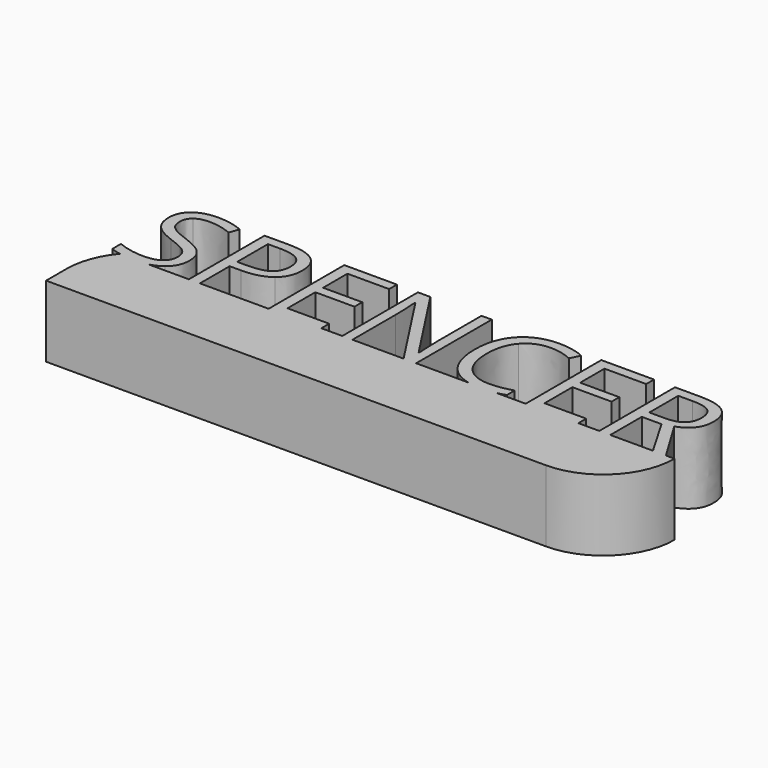
from build123d import *

# Parameters (mm, degrees)
F1_DEPTH    = 15
F2_T1_DEPTH = 63.1127871351
F2_T3_DEPTH = 90


# Not quite as in the source:
# - a fillet or chamfer that OpenCascade refuses, or shapes differently, is made with other operations: its cross-section is extruded or revolved along the edge and cut away or added


with BuildPart() as f1:
    # F0 (on Top) → F1 (new body)
    with BuildSketch(Plane.XY):
        with BuildLine():
            Line((-120, 0), (0, 0))
            Line((0, 0), (0, 15))
            Line((0, 15), (-1.8037596436, 15))
            Line((-1.8037596436, 15), (-4.5333043573, 15))
            Line((-4.5333043573, 15), (-13.4869064436, 15))
            Line((-13.4869064436, 15), (-15.7948495056, 15))
            Line((-15.7948495056, 15), (-20.1934151907, 15))
            Line((-20.1934151907, 15), (-31.2637183527, 15))
            Line((-31.2637183527, 15), (-37.436193108, 15))
            add(Edge.make_bspline(
                [(-37.436193108, 15), (-38.8938347302, 14.7261762469), (-40.691078996, 14.7261762469)],
                knots=[0.406741787, 0.406741787, 0.406741787, 1, 1, 1], degree=2))
            add(Edge.make_bspline(
                [(-40.691078996, 14.7261762469), (-42.097002764, 14.7261762469), (-43.2972236962, 15)],
                knots=[0, 0, 0, 0.3205826669, 0.3205826669, 0.3205826669], degree=2))
            Line((-43.2972236962, 15), (-54.2736064327, 15))
            Line((-54.2736064327, 15), (-56.9075301532, 15))
            Line((-56.9075301532, 15), (-67.6518526567, 15))
            Line((-67.6518526567, 15), (-69.7859393676, 15))
            Line((-69.7859393676, 15), (-74.1845050527, 15))
            Line((-74.1845050527, 15), (-85.2548082147, 15))
            Line((-85.2548082147, 15), (-99.693578181, 15))
            Line((-99.693578181, 15), (-102.0015212431, 15))
            Line((-102.0015212431, 15), (-110.5667825436, 15))
            add(Edge.make_bspline(
                [(-110.5667825436, 15), (-111.7209724053, 14.7261762469), (-113.1283277192, 14.7261762469)],
                knots=[0.5682703015, 0.5682703015, 0.5682703015, 1, 1, 1], degree=2))
            add(Edge.make_bspline(
                [(-113.1283277192, 14.7261762469), (-115.0613961391, 14.7261762469), (-116.5067974938, 15)],
                knots=[0, 0, 0, 0.5477225575, 0.5477225575, 0.5477225575], degree=2))
            Line((-116.5067974938, 15), (-120, 15))
            Line((-120, 15), (-120, 0))
        make_face()
        with BuildLine():
            Line((-4.5333043573, 15), (-1.8037596436, 15))
            Line((-1.8037596436, 15), (-7.1976529393, 23.9231772248))
            add(Edge.make_bspline(
                [(-3.2033032707, 29.24752798), (-3.2033032707, 25.3096816256), (-7.1976529393, 23.9231772248)],
                knots=[0, 0, 0, 1, 1, 1], degree=2))
            add(Edge.make_bspline(
                [(-4.9483863957, 33.4591980876), (-3.2033032707, 32.0596544605), (-3.2033032707, 29.24752798)],
                knots=[0, 0, 0, 1, 1, 1], degree=2))
            add(Edge.make_bspline(
                [(-10.3487993046, 34.8587417147), (-6.6934695208, 34.8587417147), (-4.9483863957, 33.4591980876)],
                knots=[0, 0, 0, 1, 1, 1], degree=2))
            Line((-10.3487993046, 34.8587417147), (-15.7948495056, 34.8587417147))
            Line((-15.7948495056, 34.8587417147), (-15.7948495056, 15))
            Line((-15.7948495056, 15), (-13.4869064436, 15))
            Line((-13.4869064436, 15), (-13.4869064436, 23.2581766815))
            Line((-13.4869064436, 23.2581766815), (-9.3404324677, 23.2581766815))
            Line((-9.3404324677, 23.2581766815), (-4.5333043573, 15))
        make_face()
        with BuildLine():
            Line((-10.3183744431, 25.2401390851), (-13.4869064436, 25.2401390851))
            Line((-13.4869064436, 25.2401390851), (-13.4869064436, 32.8333152233))
            Line((-13.4869064436, 32.8333152233), (-10.4835379767, 32.8333152233))
            add(Edge.make_bspline(
                [(-6.7543192437, 31.9640334673), (-7.9148103879, 32.8333152233), (-10.4835379767, 32.8333152233)],
                knots=[0, 0, 0, 1, 1, 1], degree=2))
            add(Edge.make_bspline(
                [(-5.5938280995, 29.1258285342), (-5.5938280995, 31.0947517114), (-6.7543192437, 31.9640334673)],
                knots=[0, 0, 0, 1, 1, 1], degree=2))
            add(Edge.make_bspline(
                [(-6.7347604042, 26.2115614474), (-5.5938280995, 27.1829838096), (-5.5938280995, 29.1258285342)],
                knots=[0, 0, 0, 1, 1, 1], degree=2))
            add(Edge.make_bspline(
                [(-10.3183744431, 25.2401390851), (-7.8756927089, 25.2401390851), (-6.7347604042, 26.2115614474)],
                knots=[0, 0, 0, 1, 1, 1], degree=2))
        make_face(mode=Mode.SUBTRACT)
        with BuildLine():
            add(Edge.make_bspline(
                [(-116.5067974938, 15), (-117.7003258945, 15.2261077348), (-118.5613386939, 15.6389220906)],
                knots=[0.5477225575, 0.5477225575, 0.5477225575, 1, 1, 1], degree=2))
            Line((-116.5067974938, 15), (-110.5667825436, 15))
            add(Edge.make_bspline(
                [(-107.9669672933, 16.1952624144), (-109.0475638679, 15.360424375), (-110.5667825436, 15)],
                knots=[0, 0, 0, 0.5682703015, 0.5682703015, 0.5682703015], degree=2))
            add(Edge.make_bspline(
                [(-106.0654134521, 20.2852330762), (-106.0654134521, 17.664348582), (-107.9669672933, 16.1952624144)],
                knots=[0, 0, 0, 1, 1, 1], degree=2))
            add(Edge.make_bspline(
                [(-107.2389438227, 23.5971965663), (-106.0654134521, 22.3193523851), (-106.0654134521, 20.2852330762)],
                knots=[0, 0, 0, 1, 1, 1], degree=2))
            add(Edge.make_bspline(
                [(-111.5375421058, 25.9877213952), (-108.4124741932, 24.8750407476), (-107.2389438227, 23.5971965663)],
                knots=[0, 0, 0, 1, 1, 1], degree=2))
            add(Edge.make_bspline(
                [(-114.3018580898, 27.2025426491), (-113.3978050636, 26.6527219385), (-111.5375421058, 25.9877213952)],
                knots=[0, 0, 0, 1, 1, 1], degree=2))
            add(Edge.make_bspline(
                [(-115.5862218842, 28.4130174943), (-115.2059111159, 27.7523633598), (-114.3018580898, 27.2025426491)],
                knots=[0, 0, 0, 1, 1, 1], degree=2))
            add(Edge.make_bspline(
                [(-115.9665326524, 30.1037705096), (-115.9665326524, 29.0736716288), (-115.5862218842, 28.4130174943)],
                knots=[0, 0, 0, 1, 1, 1], degree=2))
            add(Edge.make_bspline(
                [(-114.9342605672, 32.2900141258), (-115.9665326524, 31.5033141367), (-115.9665326524, 30.1037705096)],
                knots=[0, 0, 0, 1, 1, 1], degree=2))
            add(Edge.make_bspline(
                [(-112.067803977, 33.076714115), (-113.901988482, 33.076714115), (-114.9342605672, 32.2900141258)],
                knots=[0, 0, 0, 1, 1, 1], degree=2))
            add(Edge.make_bspline(
                [(-107.2867543192, 32.0466152342), (-109.7468216886, 33.076714115), (-112.067803977, 33.076714115)],
                knots=[0, 0, 0, 1, 1, 1], degree=2))
            Line((-107.2867543192, 32.0466152342), (-106.5652504618, 34.0546560904))
            add(Edge.make_bspline(
                [(-112.0113006628, 35.1412582853), (-109.0513962838, 35.1412582853), (-106.5652504618, 34.0546560904)],
                knots=[0, 0, 0, 1, 1, 1], degree=2))
            add(Edge.make_bspline(
                [(-116.577203086, 33.7830055417), (-114.8538520048, 35.1412582853), (-112.0113006628, 35.1412582853)],
                knots=[0, 0, 0, 1, 1, 1], degree=2))
            add(Edge.make_bspline(
                [(-118.3005541671, 30.1298489623), (-118.3005541671, 32.424752798), (-116.577203086, 33.7830055417)],
                knots=[0, 0, 0, 1, 1, 1], degree=2))
            add(Edge.make_bspline(
                [(-117.1118113659, 26.5853526024), (-118.3005541671, 27.9436053461), (-118.3005541671, 30.1298489623)],
                knots=[0, 0, 0, 1, 1, 1], degree=2))
            add(Edge.make_bspline(
                [(-113.1544061719, 24.236118657), (-115.9230685646, 25.2270998587), (-117.1118113659, 26.5853526024)],
                knots=[0, 0, 0, 1, 1, 1], degree=2))
            add(Edge.make_bspline(
                [(-110.2010214061, 22.9734869064), (-111.1724437683, 23.5320004346), (-113.1544061719, 24.236118657)],
                knots=[0, 0, 0, 1, 1, 1], degree=2))
            add(Edge.make_bspline(
                [(-108.8145170053, 21.7564924481), (-109.2295990438, 22.4149733782), (-110.2010214061, 22.9734869064)],
                knots=[0, 0, 0, 1, 1, 1], degree=2))
            add(Edge.make_bspline(
                [(-108.3994349669, 20.0679126372), (-108.3994349669, 21.098011518), (-108.8145170053, 21.7564924481)],
                knots=[0, 0, 0, 1, 1, 1], degree=2))
            add(Edge.make_bspline(
                [(-109.5686189286, 17.6274041074), (-108.3994349669, 18.5032054765), (-108.3994349669, 20.0679126372)],
                knots=[0, 0, 0, 1, 1, 1], degree=2))
            add(Edge.make_bspline(
                [(-113.0457459524, 16.7516027382), (-110.7378028904, 16.7516027382), (-109.5686189286, 17.6274041074)],
                knots=[0, 0, 0, 1, 1, 1], degree=2))
            add(Edge.make_bspline(
                [(-115.8969901119, 17.051504944), (-114.4583288058, 16.7516027382), (-113.0457459524, 16.7516027382)],
                knots=[0, 0, 0, 1, 1, 1], degree=2))
            add(Edge.make_bspline(
                [(-118.5613386939, 17.8642833859), (-117.335651418, 17.3514071498), (-115.8969901119, 17.051504944)],
                knots=[0, 0, 0, 1, 1, 1], degree=2))
            Line((-118.5613386939, 17.8642833859), (-118.5613386939, 15.6389220906))
        make_face()
        with BuildLine():
            Line((-110.5667825436, 15), (-116.5067974938, 15))
            add(Edge.make_bspline(
                [(-113.1283277192, 14.7261762469), (-115.0613961391, 14.7261762469), (-116.5067974938, 15)],
                knots=[0, 0, 0, 0.5477225575, 0.5477225575, 0.5477225575], degree=2))
            add(Edge.make_bspline(
                [(-110.5667825436, 15), (-111.7209724053, 14.7261762469), (-113.1283277192, 14.7261762469)],
                knots=[0.5682703015, 0.5682703015, 0.5682703015, 1, 1, 1], degree=2))
        make_face()
        with BuildLine():
            Line((-102.0015212431, 34.8587417147), (-102.0015212431, 15))
            Line((-102.0015212431, 15), (-99.693578181, 15))
            Line((-99.693578181, 15), (-99.693578181, 22.8104965772))
            Line((-99.693578181, 22.8104965772), (-97.3552102575, 22.8104965772))
            add(Edge.make_bspline(
                [(-91.4679995654, 24.4338802564), (-93.5260241226, 22.8104965772), (-97.3552102575, 22.8104965772)],
                knots=[0, 0, 0, 1, 1, 1], degree=2))
            add(Edge.make_bspline(
                [(-89.4099750081, 29.0736716288), (-89.4099750081, 26.0572639357), (-91.4679995654, 24.4338802564)],
                knots=[0, 0, 0, 1, 1, 1], degree=2))
            add(Edge.make_bspline(
                [(-96.8510268391, 34.8587417147), (-89.4099750081, 34.8587417147), (-89.4099750081, 29.0736716288)],
                knots=[0, 0, 0, 1, 1, 1], degree=2))
            Line((-96.8510268391, 34.8587417147), (-102.0015212431, 34.8587417147))
        make_face()
        with BuildLine():
            Line((-97.6116483755, 24.7924589808), (-99.693578181, 24.7924589808))
            Line((-99.693578181, 24.7924589808), (-99.693578181, 32.859393676))
            Line((-99.693578181, 32.859393676), (-97.1118113659, 32.859393676))
            add(Edge.make_bspline(
                [(-93.0913832446, 31.8966641313), (-94.3822666522, 32.859393676), (-97.1118113659, 32.859393676)],
                knots=[0, 0, 0, 1, 1, 1], degree=2))
            add(Edge.make_bspline(
                [(-91.800499837, 28.9650114093), (-91.800499837, 30.9339345865), (-93.0913832446, 31.8966641313)],
                knots=[0, 0, 0, 1, 1, 1], degree=2))
            add(Edge.make_bspline(
                [(-93.171791807, 25.7834401825), (-91.800499837, 26.7744213843), (-91.800499837, 28.9650114093)],
                knots=[0, 0, 0, 1, 1, 1], degree=2))
            add(Edge.make_bspline(
                [(-97.6116483755, 24.7924589808), (-94.543083777, 24.7924589808), (-93.171791807, 25.7834401825)],
                knots=[0, 0, 0, 1, 1, 1], degree=2))
        make_face(mode=Mode.SUBTRACT)
        Polygon((-31.2637183527, 15), (-20.1934151907, 15), (-20.1934151907, 17.0645441704), (-28.9557752907, 17.0645441704), (-28.9557752907, 24.3708573291), (-20.7236770618, 24.3708573291), (-20.7236770618, 26.4093230468), (-28.9557752907, 26.4093230468), (-28.9557752907, 32.8072367706), (-20.1934151907, 32.8072367706), (-20.1934151907, 34.8587417147), (-31.2637183527, 34.8587417147), align=None)
        Polygon((-85.2548082147, 34.8587417147), (-85.2548082147, 15), (-74.1845050527, 15), (-74.1845050527, 17.0645441704), (-82.9468651527, 17.0645441704), (-82.9468651527, 24.3708573291), (-74.7147669238, 24.3708573291), (-74.7147669238, 26.4093230468), (-82.9468651527, 26.4093230468), (-82.9468651527, 32.8072367706), (-74.1845050527, 32.8072367706), (-74.1845050527, 34.8587417147), align=None)
        with BuildLine():
            add(Edge.make_bspline(
                [(-37.436193108, 15), (-38.8938347302, 14.7261762469), (-40.691078996, 14.7261762469)],
                knots=[0.406741787, 0.406741787, 0.406741787, 1, 1, 1], degree=2))
            Line((-37.436193108, 15), (-43.2972236962, 15))
            add(Edge.make_bspline(
                [(-40.691078996, 14.7261762469), (-42.097002764, 14.7261762469), (-43.2972236962, 15)],
                knots=[0, 0, 0, 0.3205826669, 0.3205826669, 0.3205826669], degree=2))
        make_face()
        with BuildLine():
            Line((-43.2972236962, 15), (-37.436193108, 15))
            add(Edge.make_bspline(
                [(-35.5970879061, 15.5041834185), (-36.4368242914, 15.1877353912), (-37.436193108, 15)],
                knots=[0, 0, 0, 0.406741787, 0.406741787, 0.406741787], degree=2))
            Line((-35.5970879061, 15.5041834185), (-35.5970879061, 17.525263501))
            add(Edge.make_bspline(
                [(-40.3390198848, 16.7776811909), (-38.2614364881, 16.7776811909), (-35.5970879061, 17.525263501)],
                knots=[0, 0, 0, 1, 1, 1], degree=2))
            add(Edge.make_bspline(
                [(-45.5481908073, 18.9052482886), (-43.7205259155, 16.7776811909), (-40.3390198848, 16.7776811909)],
                knots=[0, 0, 0, 1, 1, 1], degree=2))
            add(Edge.make_bspline(
                [(-47.3758556992, 24.9271976529), (-47.3758556992, 21.0328153863), (-45.5481908073, 18.9052482886)],
                knots=[0, 0, 0, 1, 1, 1], degree=2))
            add(Edge.make_bspline(
                [(-45.4808214713, 30.8969901119), (-47.3758556992, 28.7172661089), (-47.3758556992, 24.9271976529)],
                knots=[0, 0, 0, 1, 1, 1], degree=2))
            add(Edge.make_bspline(
                [(-40.3129414321, 33.076714115), (-43.5857872433, 33.076714115), (-45.4808214713, 30.8969901119)],
                knots=[0, 0, 0, 1, 1, 1], degree=2))
            add(Edge.make_bspline(
                [(-35.8013691188, 32.0205367815), (-38.0571552755, 33.076714115), (-40.3129414321, 33.076714115)],
                knots=[0, 0, 0, 1, 1, 1], degree=2))
            Line((-35.8013691188, 32.0205367815), (-34.8234271433, 34.002499185))
            add(Edge.make_bspline(
                [(-40.2825165707, 35.1412582853), (-37.1617950668, 35.1412582853), (-34.8234271433, 34.002499185)],
                knots=[0, 0, 0, 1, 1, 1], degree=2))
            add(Edge.make_bspline(
                [(-45.3830272737, 33.8916657612), (-43.216342497, 35.1412582853), (-40.2825165707, 35.1412582853)],
                knots=[0, 0, 0, 1, 1, 1], degree=2))
            add(Edge.make_bspline(
                [(-48.6971639683, 30.3341301749), (-47.5497120504, 32.642073237), (-45.3830272737, 33.8916657612)],
                knots=[0, 0, 0, 1, 1, 1], degree=2))
            add(Edge.make_bspline(
                [(-49.8446158861, 24.9576225144), (-49.8446158861, 28.0261871129), (-48.6971639683, 30.3341301749)],
                knots=[0, 0, 0, 1, 1, 1], degree=2))
            add(Edge.make_bspline(
                [(-47.4606106704, 17.3905248289), (-49.8446158861, 20.0548734108), (-49.8446158861, 24.9576225144)],
                knots=[0, 0, 0, 1, 1, 1], degree=2))
            add(Edge.make_bspline(
                [(-43.2972236962, 15), (-45.8408762047, 15.5803202209), (-47.4606106704, 17.3905248289)],
                knots=[0.3205826669, 0.3205826669, 0.3205826669, 1, 1, 1], degree=2))
        make_face()
        with BuildLine():
            Line((-69.7859393676, 34.8587417147), (-69.7859393676, 15))
            Line((-69.7859393676, 15), (-67.6518526567, 15))
            Line((-67.6518526567, 15), (-67.6518526567, 26.287623601))
            add(Edge.make_bspline(
                [(-67.8691730957, 31.6641312615), (-67.6518526567, 28.7303053352), (-67.6518526567, 26.287623601)],
                knots=[0, 0, 0, 1, 1, 1], degree=2))
            Line((-67.8691730957, 31.6641312615), (-67.7605128762, 31.6641312615))
            Line((-67.7605128762, 31.6641312615), (-56.9075301532, 15))
            Line((-56.9075301532, 15), (-54.2736064327, 15))
            Line((-54.2736064327, 15), (-54.2736064327, 34.8587417147))
            Line((-54.2736064327, 34.8587417147), (-56.4337715962, 34.8587417147))
            Line((-56.4337715962, 34.8587417147), (-56.4337715962, 23.4624578942))
            add(Edge.make_bspline(
                [(-56.3642290557, 20.6155601434), (-56.4598500489, 22.6062153646), (-56.4337715962, 23.4624578942)],
                knots=[0, 0, 0, 1, 1, 1], degree=2))
            add(Edge.make_bspline(
                [(-56.2425296099, 18.2598065848), (-56.2686080626, 18.6249049223), (-56.3642290557, 20.6155601434)],
                knots=[0, 0, 0, 1, 1, 1], degree=2))
            Line((-56.2425296099, 18.2598065848), (-56.3511898294, 18.2598065848))
            Line((-56.3511898294, 18.2598065848), (-67.1780940998, 34.8587417147))
            Line((-67.1780940998, 34.8587417147), (-69.7859393676, 34.8587417147))
        make_face()
    extrude(amount=F1_DEPTH)

    # F2: fillet of radius 15 on 2 edges, made by hand

    # F2_s2 → F2_t1 (cut)
    with BuildSketch(Plane.XY.offset(-24.0563935676)):
        with BuildLine():
            ThreePointArc((-116.5067974938, 15), (-119.0996801809, 10.4959402819), (-120, 5.377442573))
            Line((-120, 5.377442573), (-120, 15))
            Line((-120, 15), (-116.5067974938, 15))
        make_face()
    extrude(amount=F2_T1_DEPTH, mode=Mode.SUBTRACT)

    # F2_s4 → F2_t3 (cut)
    with BuildSketch(Plane.XY.offset(-37.5)):
        with BuildLine():
            ThreePointArc((-15, 0), (-4.3933982822, 4.3933982822), (0, 15))
            Line((0, 15), (0, 0))
            Line((0, 0), (-15, 0))
        make_face()
    extrude(amount=F2_T3_DEPTH, mode=Mode.SUBTRACT)


solid = f1.part
